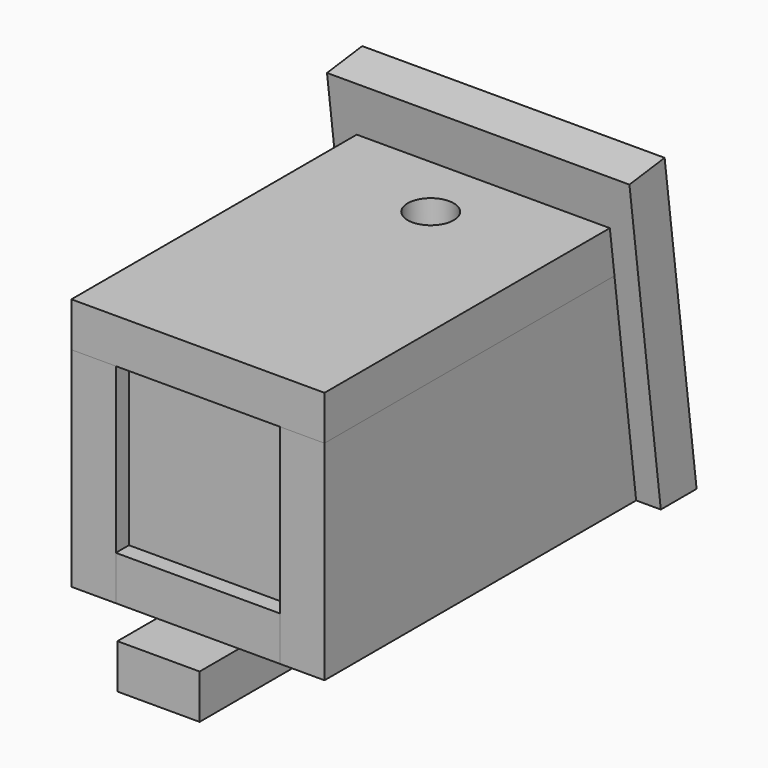
from build123d import *

# Parameters (mm, degrees)
F0_W      = 100
F0_H      = 237
F1_DEPTH  = 27
F2_W      = 100
F2_H      = 27
F3_DEPTH  = 100
F4_W      = 27
F4_H      = 100
F4_W_2    = 200
F4_W_3    = 10
F5_DEPTH  = 27
F6_W      = 27
F6_H      = 237
F6_W_2    = 127
F7_DEPTH  = 27
F8_R      = 14
F9_DEPTH  = 27
F11_DEPTH = 154.001
F13_DEPTH = 27
F14_W     = 100
F14_H     = 27.2267423081
F14_H_2   = 100.8397863263
F15_DEPTH = 27
F17_DEPTH = 184
F18_W     = 50
F18_H     = 30
F18_H_2   = 237
F18_H_3   = 27.2267423081
F19_DEPTH = 27


with BuildPart() as f1:
    # F0 (on Top) → F1 (new body)
    with BuildSketch(Plane.XY):
        with Locations((50, 118.5)):
            Rectangle(F0_W, F0_H)
    extrude(amount=F1_DEPTH)


with BuildPart() as f3:
    # F2 (on face) → F3 (new body)
    with BuildSketch(Plane.XY.offset(27)):
        with Locations((50, 23.5)):
            Rectangle(F2_W, F2_H)
    extrude(amount=F3_DEPTH)


with BuildPart() as f5:
    # F4 (on face) → F5 (new body)
    with BuildSketch(Plane.YZ.offset(100)):
        with Locations((23.5, 77)):
            Rectangle(F4_W, F4_H)
        with Locations((137, 77)):
            Rectangle(F4_W_2, F4_H)
        Polygon((0, 27), (0, 0), (237, 0), (237, 27), (37, 27), (10, 27), align=None)
        with Locations((5, 77)):
            Rectangle(F4_W_3, F4_H)
    extrude(amount=F5_DEPTH)


with BuildPart() as f7:
    # F6 (on face) → F7 (new body)
    with BuildSketch(Plane.XY.offset(127)):
        with Locations((113.5, 118.5)):
            Rectangle(F6_W, F6_H)
        with Locations((36.5, 118.5)):
            Rectangle(F6_W_2, F6_H)
    extrude(amount=F7_DEPTH)

    # F8 (on face) → F9 (cut, through all)
    with BuildSketch(Plane.XY.offset(154)):
        with Locations((50, 177)):
            Circle(F8_R)
    extrude(amount=-F9_DEPTH, mode=Mode.SUBTRACT)


with BuildPart() as f11_tool:
    # F10 (on face) → F11 (new body, through all)
    with BuildSketch(Plane.YZ.offset(127)):
        Polygon((237, 127), (220.5064935065, 127), (237, 0), align=None)
        Polygon((217, 154), (220.5064935065, 127), (237, 127), (237, 154), align=None)
    extrude(amount=-F11_DEPTH)


with BuildPart() as f1_1:
    add(f1.part)

    # F11: cut by f11_tool
    add(f11_tool.part, mode=Mode.SUBTRACT)


with BuildPart() as f5_1:
    add(f5.part)

    # F11: cut by f11_tool
    add(f11_tool.part, mode=Mode.SUBTRACT)


with BuildPart() as f7_1:
    add(f7.part)

    # F11: cut by f11_tool
    add(f11_tool.part, mode=Mode.SUBTRACT)


with BuildPart() as f13:
    # F12 (on face) → F13 (new body)
    with BuildSketch(Plane(origin=(0, 0, 0), x_dir=(0, -1, 0), z_dir=(-1, 0, 0))):
        Polygon((0, 127), (-220.5064935065, 127), (-233.4935064935, 27), (0, 27), align=None)
        Polygon((0, 27), (-233.4935064935, 27), (-237, 0), (0, 0), align=None)
    extrude(amount=F13_DEPTH)


with BuildPart() as f15:
    # F14 (on face) → F15 (new body)
    with BuildSketch(Plane(origin=(0, 233.0689998341, 30.2687012772), x_dir=(-1, 0, 0), z_dir=(0, 0.9916720735, 0.128788581))):
        Polygon((27, -30.5228936916), (27, 97.5436349427), (0, 97.5436349427), (0, -3.2961513835), (0, -30.5228936916), align=None)
        Polygon((27, 124.7703772508), (27, 97.5436349427), (27, -30.5228936916), (42, -30.5228936916), (42, 154.7703772508), (-142, 154.7703772508), (-142, -30.5228936916), (-127, -30.5228936916), (-127, 97.5436349427), (-127, 124.7703772508), align=None)
        Polygon((-100, -3.2961513835), (-100, 97.5436349427), (-127, 97.5436349427), (-127, -30.5228936916), (-100, -30.5228936916), align=None)
        with Locations((-50, -16.9095225376)):
            Rectangle(F14_W, F14_H)
        Polygon((0, 97.5436349427), (27, 97.5436349427), (27, 124.7703772508), (-127, 124.7703772508), (-127, 97.5436349427), (-100, 97.5436349427), align=None)
        with Locations((-50, 47.1237417796)):
            Rectangle(F14_W, F14_H_2)
    extrude(amount=F15_DEPTH)

    # F16 (on face) → F17 (join, through all)
    with BuildSketch(Plane(origin=(-42, 0, 0), x_dir=(0, -1, 0), z_dir=(-1, 0, 0))):
        Polygon((-264.2267423081, 0), (-237, 0), (-263.7751459852, 3.4772916864), align=None)
    extrude(amount=-F17_DEPTH)


with BuildPart() as f19:
    # F18 (on face) → F19 (new body)
    with BuildSketch(Plane(origin=(0, 0, 0), x_dir=(1, 0, 0), z_dir=(0, 0, -1))):
        with Locations((50, 15)):
            Rectangle(F18_W, F18_H)
        with Locations((50, -118.5)):
            Rectangle(F18_W, F18_H_2)
        with Locations((50, -250.613371154)):
            Rectangle(F18_W, F18_H_3)
        with Locations((50, -279.2267423081)):
            Rectangle(F18_W, F18_H)
    extrude(amount=F19_DEPTH)


solid = Compound([f3.part, f1_1.part, f5_1.part, f7_1.part, f13.part, f15.part, f19.part])
